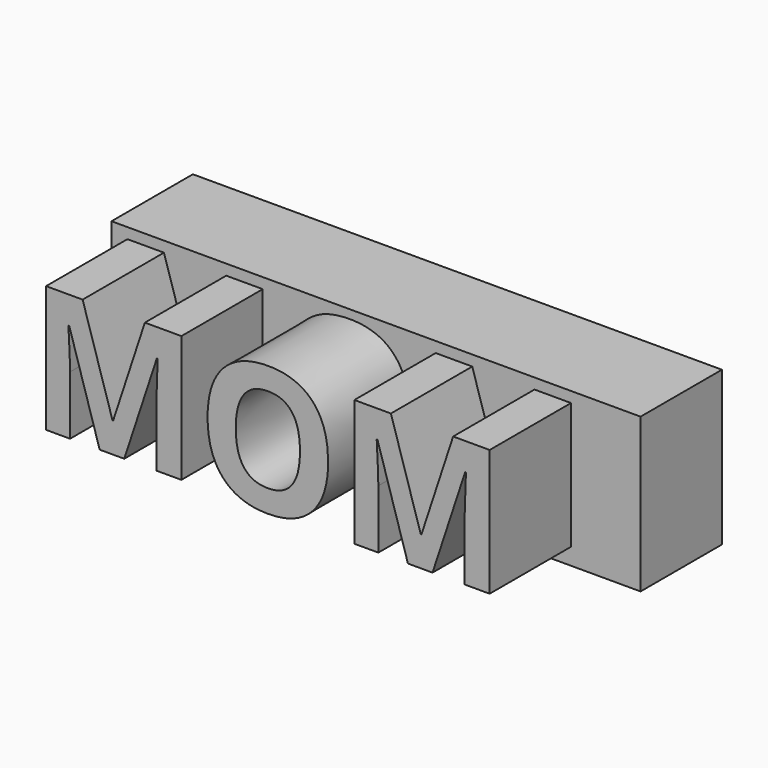
from build123d import *

# Parameters (mm, degrees)
F0_W         = 81.3509523869
F0_H         = 38.440560922
F1_DEPTH     = 25.4
F2_TEXT_SIZE = 44.2844518046
F3_DEPTH     = 25.4
F4_DEPTH     = 25.4
F5_DEPTH     = 25.4


# Not quite as in the source:
# - Text() gives the source's letters only with a copy of the font that has no kerning and outlines rounded to 1/6400 em; it was checked with that copy


with BuildPart() as f1:
    # F0 (on Front) → F1 (new body)
    with BuildSketch(Plane.XZ):
        with Locations((3.1288824975, 1.787933521)):
            Rectangle(F0_W, F0_H)
    extrude(amount=F1_DEPTH)

    # F2 (on face) → F3 (join)
    with BuildSketch(Plane.XZ.offset(25.4)):
        with Locations((-37.5465936959, -13.2605032995)):
            Text('MOM', F2_TEXT_SIZE, font='Open Sans', font_style=FontStyle.BOLD, text_align=(TextAlign.LEFT, TextAlign.BOTTOM))
    extrude(amount=F3_DEPTH)

    # F4 (add): a face of the model
    f4_faces = [f1.faces().sort_by_distance(p)[0] for p in [
        (43.804358691, -12.7, 1.787933521),
    ]]
    extrude(f4_faces, amount=F4_DEPTH)

    # F5 (add): a face of the model
    f5_faces = [f1.faces().sort_by_distance(p)[0] for p in [
        (69.204358691, -12.7, 1.787933521),
    ]]
    extrude(f5_faces, amount=F5_DEPTH)


solid = f1.part
